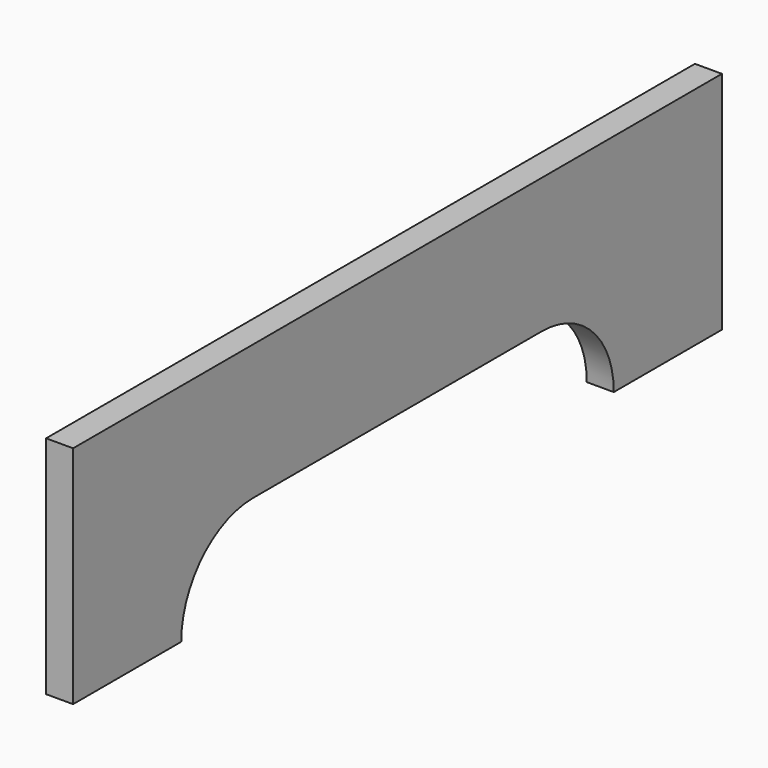
from build123d import *

# Parameters (mm, degrees)
F0_W     = 180
F0_H     = 50
F1_DEPTH = 6
F2_W     = 120
F2_H     = 20
F3_DEPTH = 25
F4_R     = 19.99999


# Not quite as in the source:
# - a fillet or chamfer is up to 0.001 mm smaller than in the source, because OpenCascade refuses the exact size


with BuildPart() as f1:
    # F0 (on Right) → F1 (new body)
    with BuildSketch(Plane.YZ):
        Rectangle(F0_W, F0_H)
    extrude(amount=F1_DEPTH)

    # F2 (on face) → F3 (cut)
    with BuildSketch(Plane.YZ.offset(6)):
        with Locations((0, -15)):
            Rectangle(F2_W, F2_H)
    extrude(amount=-F3_DEPTH, mode=Mode.SUBTRACT)

    # F4 (radius 20 in the source; OpenCascade refuses exactly that, so slightly less here)
    f4_edges = [f1.edges().sort_by_distance(p)[0] for p in [
        (3, 60, -5),
        (3, -60, -5),
    ]]
    fillet(f4_edges, radius=F4_R)


solid = f1.part
